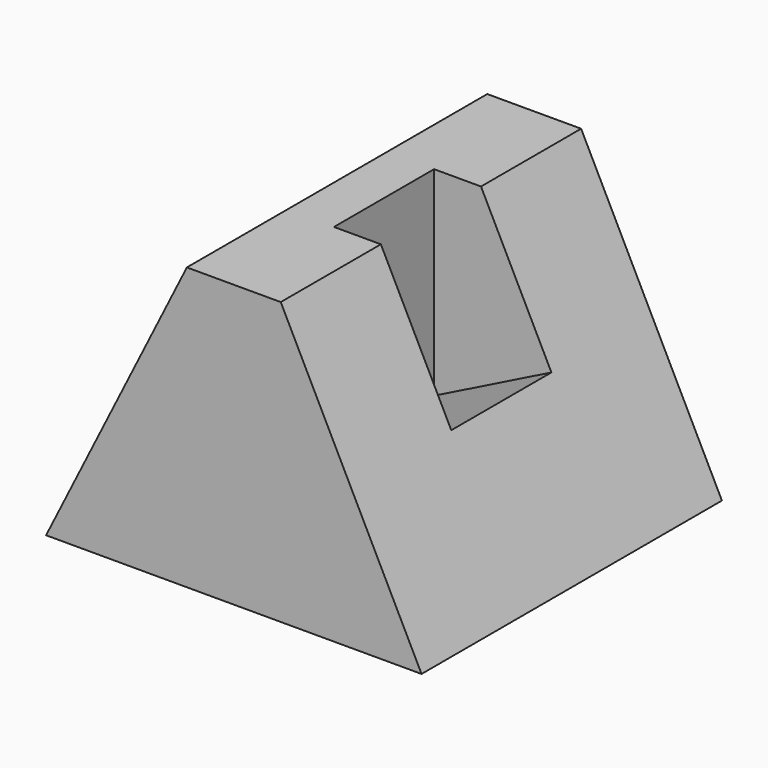
from build123d import *

# Parameters (mm, degrees)
F1_DEPTH = 20
F2_DEPTH = 6.6666666667


# Not quite as in the source:
# - a feature names something its author has since deleted; it is built from what else it names


with BuildPart() as f1:
    # F0 (on Front) → F1 (new body, symmetric)
    with BuildSketch(Plane.XZ):
        Polygon((15, 30), (0, 0), (40, 0), (32.5, 15), (20, 8.75), (20, 30), align=None)
        Polygon((20, 8.75), (32.5, 15), (25, 30), (20, 30), align=None)
    extrude(amount=F1_DEPTH, both=True)

    # F0 (on Front) → F2 (cut, symmetric)
    with BuildSketch(Plane.XZ):
        Polygon((20, 8.75), (32.5, 15), (25, 30), (20, 30), align=None)
    extrude(amount=F2_DEPTH, both=True, mode=Mode.SUBTRACT)


solid = f1.part
